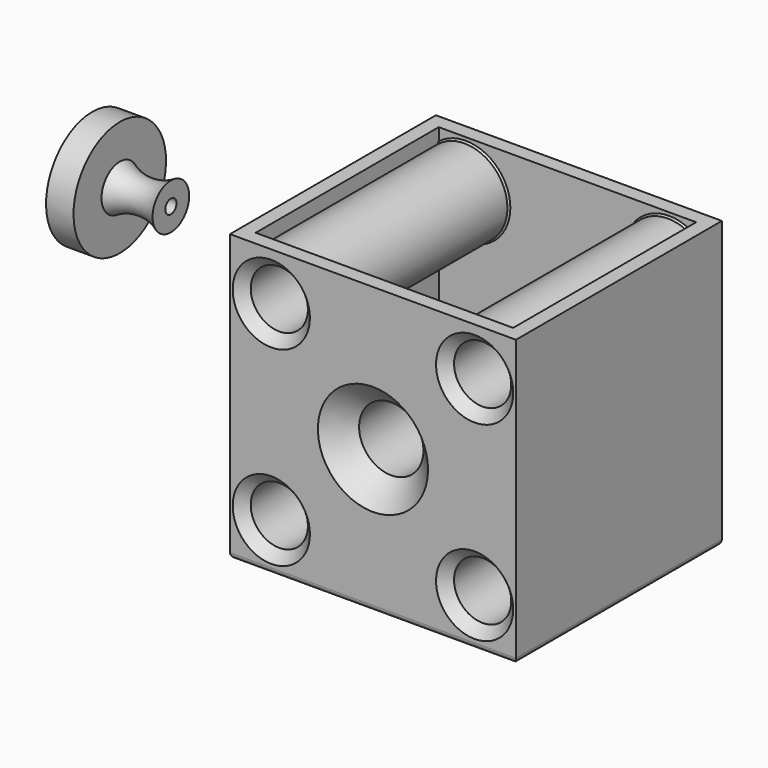
from build123d import *

# Parameters (mm, degrees)
F0_W     = 127
F0_H     = 127
F0_R     = 12.7
F0_R_2   = 14.2875
F1_DEPTH = 114.3
F2_R     = 2.54
F3_SIZE  = 4.445
F4_SIZE  = 10.16
F5_T     = 6.35
F8_R     = 3.112849
F9_DEPTH = 42.638296021


# Not quite as in the source:
# - a shell that OpenCascade refuses in one call is made with other operations: the cavity is built on its own and cut out


with BuildPart() as f1:
    # F0 (on Front) → F1 (new body)
    with BuildSketch(Plane.XZ):
        with Locations((-9.5917450488, -27.3068194985)):
            Rectangle(F0_W, F0_H)
        with Locations((-54.7332502902, -69.6027859598)):
            Circle(F0_R, mode=Mode.SUBTRACT)
        with Locations((35.5497601926, -69.6027859598)):
            Circle(F0_R, mode=Mode.SUBTRACT)
        with Locations((-54.7332502902, 14.9891469628)):
            Circle(F0_R, mode=Mode.SUBTRACT)
        with Locations((-9.5917450488, -27.3068194985)):
            Circle(F0_R_2, mode=Mode.SUBTRACT)
        with Locations((35.5497601926, 14.9891469628)):
            Circle(F0_R, mode=Mode.SUBTRACT)
    extrude(amount=-F1_DEPTH)

    # F2
    f2_edges = [f1.edges().sort_by_distance(p)[0] for p in [
        (53.908255, 57.15, -90.806819),
        (-9.591745, 0, -90.806819),
        (-9.591745, 114.3, -90.806819),
        (-73.091745, 57.15, -90.806819),
    ]]
    fillet(f2_edges, radius=F2_R)

    # F3
    f3_edges = [f1.edges().sort_by_distance(p)[0] for p in [
        (-67.43325, 0, 14.989147),
        (-67.43325, 0, -69.602786),
        (22.84976, 0, -69.602786),
        (22.84976, 0, 14.989147),
        (22.84976, 114.3, 14.989147),
        (-67.43325, 114.3, 14.989147),
        (-23.879245, 114.3, -27.306819),
        (22.84976, 114.3, -69.602786),
        (-67.43325, 114.3, -69.602786),
    ]]
    chamfer(f3_edges, length=F3_SIZE)

    # F4
    f4_edges = [f1.edges().sort_by_distance(p)[0] for p in [
        (-23.879245, 0, -27.306819),
    ]]
    chamfer(f4_edges, length=F4_SIZE)

    # F5: shell of thickness 6.35, made by hand


with BuildPart() as f5_core1:
    # F5_t2: copy of F1
    add(f1.part)

    # the walls: a layer under each face that stays
    f5_faces = [f5_core1.faces().sort_by_distance(p)[0] for p in [
        (-51.9250783821, 0, -26.0368194985),
        (-28.9592450488, 5.08, -27.3068194985),
        (-69.6557502902, 2.2225, 14.9891469628),
        (-73.0917450488, 57.15, -26.0368194985),
        (53.9082549512, 57.15, -26.0368194985),
        (-69.6557502902, 2.2225, -69.6027859598),
        (20.6272601926, 2.2225, -69.6027859598),
        (20.6272601926, 2.2225, 14.9891469628),
        (-23.8792450488, 60.0075, -27.3068194985),
        (-67.4332502902, 57.15, 14.9891469628),
        (-51.9250783821, 114.3, -26.0368194985),
        (-9.5917450488, 57.15, -90.8068194985),
        (-67.4332502902, 57.15, -69.6027859598),
        (22.8497601926, 57.15, -69.6027859598),
        (22.8497601926, 57.15, 14.9891469628),
        (-26.1017450488, 112.0775, -27.3068194985),
        (-69.6557502902, 112.0775, 14.9891469628),
        (20.6272601926, 112.0775, 14.9891469628),
        (20.6272601926, 112.0775, -69.6027859598),
        (-69.6557502902, 112.0775, -69.6027859598),
    ]]
    thicken(f5_faces, amount=-F5_T, mode=Mode.SUBTRACT)


with BuildPart() as f1_1:
    add(f1.part)

    # what is left inside the walls is the cavity
    f5_cavity = [f5_core1.part.solids().sort_by_distance(p)[0] for p in [
        (-30.292745, 75.746581, -27.306819),
        (47.557589, 73.841581, -84.473493),
        (-66.741079, 73.841581, -84.473493),
    ]]
    add(f5_cavity, mode=Mode.SUBTRACT)


with BuildPart() as f7:
    # F6 (on Front) → F7 (revolve)
    with BuildSketch(Plane.XZ):
        with BuildLine():
            Line((-141.9669985771, 48.6336536705), (-141.9669985771, 38.4819172323))
            Line((-141.9669985771, 38.4819172323), (-99.3297025561, 38.4819172323))
            Line((-99.3297025561, 38.4819172323), (-99.3297025561, 48.6336536705))
            ThreePointArc((-99.3297025561, 48.6336536705), (-110.6663122773, 45.4203041339), (-122.0029219985, 48.6336536705))
            Line((-122.0029219985, 48.6336536705), (-122.0029219985, 64.1448497772))
            Line((-122.0029219985, 64.1448497772), (-134.2117935419, 64.1448497772))
            Line((-134.2117935419, 64.1448497772), (-134.2117935419, 48.6336536705))
            Line((-134.2117935419, 48.6336536705), (-136.32799685, 55.8428168297))
            Line((-136.32799685, 55.8428168297), (-141.9669985771, 48.6336536705))
        make_face()
    revolve(axis=Axis((-120.6483505666, 0, 38.4819172323), (1, 0, 0)))

    # F8 (on face) → F9 (cut, through all)
    with BuildSketch(Plane.YZ.offset(-99.3297025561)):
        with Locations((0, 38.4819172323)):
            Circle(F8_R)
    extrude(amount=-F9_DEPTH, mode=Mode.SUBTRACT)


solid = Compound([f1_1.part, f7.part])
